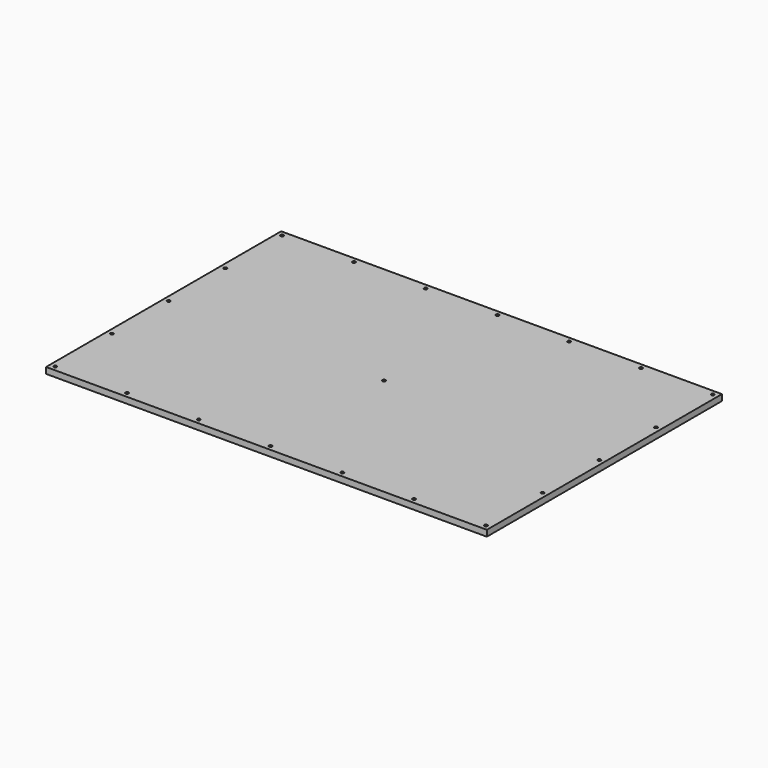
from build123d import *

# Parameters (mm, degrees)
F1_W     = 457.2
F1_H     = 304.8
F2_DEPTH = 6.35
F4_D     = 3.3


# Not quite as in the source:
# - a variable given as a bare number and used for a length is read in inches; the dataset says mm whatever the document's units were


with BuildPart() as f2:
    # F1 (on Top) → F2 (new body)
    with BuildSketch(Plane.XY):
        Rectangle(F1_W, F1_H)
    extrude(amount=F2_DEPTH)

    # F4 (through all)
    with Locations(Plane.XY.offset(6.35)):
        with Locations((-223.3168, 147.1168), (-148.8778666667, 147.1168), (-74.4389333333, 147.1168), (0, 147.1168), (74.4389333333, 147.1168), (148.8778666667, 147.1168), (223.3168, 147.1168), (223.3168, 73.5584), (223.3168, 0), (223.3168, -73.5584), (223.3168, -147.1168), (148.8778666667, -147.1168), (74.4389333333, -147.1168), (0, -147.1168), (-74.4389333333, -147.1168), (-148.8778666667, -147.1168), (-223.3168, -73.5584), (-223.3168, -147.1168), (-223.3168, 0), (-223.3168, 73.5584), (0, 0)):
            Hole(F4_D / 2)


solid = f2.part
